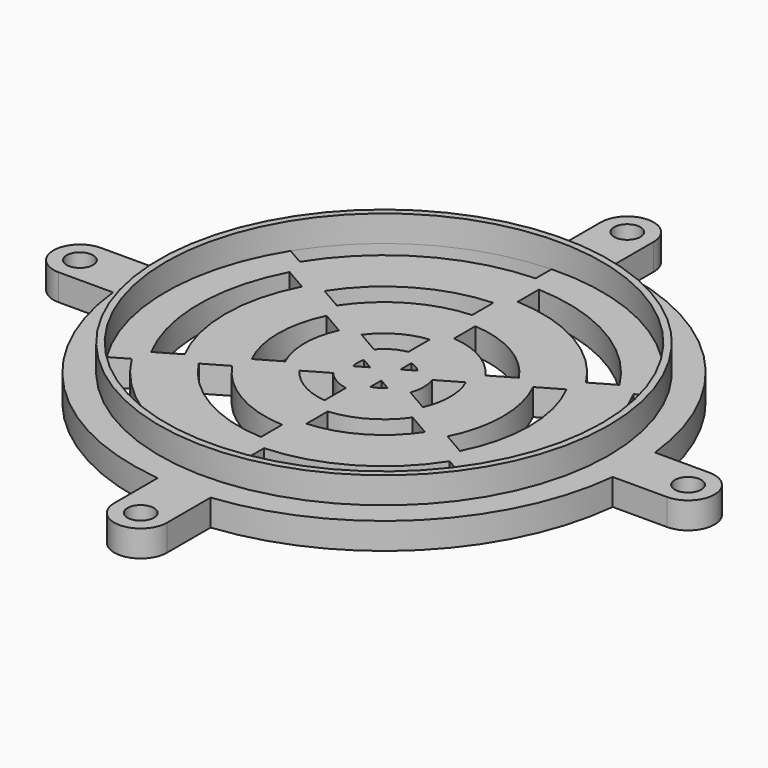
from build123d import *

# Parameters (mm, degrees)
F0_R     = 1.5875
F1_DEPTH = 3.175
F2_R     = 26.9875
F2_R_2   = 26.19375
F3_DEPTH = 3.175
F5_DEPTH = 3.175


# Not quite as in the source:
# - after a boolean that leaves OpenCascade's solid faulty, fix() repairs it


with BuildPart() as f1:
    # F0 (on Top) → F1 (new body)
    with BuildSketch(Plane.XY):
        with BuildLine():
            Line((36.5125, 3.175), (29.994929259, 3.175))
            ThreePointArc((29.994929259, 3.175), (21.3281082875, 21.3281082875), (3.175, 29.994929259))
            Line((3.175, 29.994929259), (3.175, 36.5125))
            ThreePointArc((3.175, 36.5125), (0, 39.6875), (-3.175, 36.5125))
            Line((-3.175, 36.5125), (-3.175, 29.994929259))
            ThreePointArc((-3.175, 29.994929259), (-21.3281082875, 21.3281082875), (-29.994929259, 3.175))
            Line((-29.994929259, 3.175), (-30.1625, 3.175))
            Line((-30.1625, 3.175), (-36.5125, 3.175))
            ThreePointArc((-36.5125, 3.175), (-39.6875, 0), (-36.5125, -3.175))
            Line((-36.5125, -3.175), (-30.1625, -3.175))
            Line((-30.1625, -3.175), (-29.994929259, -3.175))
            ThreePointArc((-29.994929259, -3.175), (-21.3281082875, -21.3281082875), (-3.175, -29.994929259))
            Line((-3.175, -29.994929259), (-3.175, -36.5125))
            ThreePointArc((-3.175, -36.5125), (0, -39.6875), (3.175, -36.5125))
            Line((3.175, -36.5125), (3.175, -29.994929259))
            ThreePointArc((3.175, -29.994929259), (21.3281082875, -21.3281082875), (29.994929259, -3.175))
            Line((29.994929259, -3.175), (36.5125, -3.175))
            ThreePointArc((36.5125, -3.175), (39.6875, 0), (36.5125, 3.175))
        make_face()
        with Locations((0, -36.5125)):
            Circle(F0_R, mode=Mode.SUBTRACT)
        with Locations((-36.5125, 0)):
            Circle(F0_R, mode=Mode.SUBTRACT)
        with Locations((36.5125, 0)):
            Circle(F0_R, mode=Mode.SUBTRACT)
        with Locations((0, 36.5125)):
            Circle(F0_R, mode=Mode.SUBTRACT)
    extrude(amount=F1_DEPTH)

    # F2 (on face) → F3 (join)
    with BuildSketch(Plane.XY.offset(3.175)):
        Circle(F2_R)
        Circle(F2_R_2, mode=Mode.SUBTRACT)
    extrude(amount=F3_DEPTH)

    # F4 (on face) → F5 (cut)
    with BuildSketch(Plane.XY.offset(3.175)):
        with BuildLine():
            ThreePointArc((-0.8255, 26.1807388897), (-13.096875, 22.6844529204), (-22.2604349684, 13.8052734157))
            Line((-22.2604349684, 13.8052734157), (-20.1970845335, 12.6139974867))
            ThreePointArc((-20.1970845335, 12.6139974867), (-11.90625, 20.6222299276), (-0.8255, 23.7981870318))
            Line((-0.8255, 23.7981870318), (-0.8255, 26.1807388897))
        make_face()
        with BuildLine():
            ThreePointArc((0.8255, 19.0321057624), (9.525, 16.4977839421), (16.0695370777, 10.230956852))
            Line((16.0695370777, 10.230956852), (18.8213832288, 11.8197359681))
            ThreePointArc((18.8213832288, 11.8197359681), (11.1125, 19.2474145991), (0.8255, 22.2096639945))
            Line((0.8255, 22.2096639945), (0.8255, 19.0321057624))
        make_face()
        with BuildLine():
            Line((21.0225845335, -11.1841895451), (23.0859349684, -12.375465474))
            ThreePointArc((23.0859349684, -12.375465474), (25.4049183047, -6.3798640262), (26.19375, 0))
            ThreePointArc((26.19375, 0), (25.4049183047, 6.3798640262), (23.0859349684, 12.375465474))
            Line((23.0859349684, 12.375465474), (21.0225845335, 11.1841895451))
            ThreePointArc((21.0225845335, 11.1841895451), (23.8125, 0), (21.0225845335, -11.1841895451))
        make_face()
        with BuildLine():
            Line((12.7654179102, -6.4169121723), (15.5188114324, -8.0065846636))
            ThreePointArc((15.5188114324, -8.0065846636), (17.4625, 0), (15.5188114324, 8.0065846636))
            Line((15.5188114324, 8.0065846636), (12.7654179102, 6.4169121723))
            ThreePointArc((12.7654179102, 6.4169121723), (14.2875, 0), (12.7654179102, -6.4169121723))
        make_face()
        with BuildLine():
            Line((4.4747651403, -1.6303015639), (7.2495505675, -3.2323246772))
            ThreePointArc((7.2495505675, -3.2323246772), (7.9375, 0), (7.2495505675, 3.2323246772))
            Line((7.2495505675, 3.2323246772), (4.4747651403, 1.6303015639))
            ThreePointArc((4.4747651403, 1.6303015639), (4.7625, 0), (4.4747651403, -1.6303015639))
        make_face()
        with BuildLine():
            ThreePointArc((0.8255, 9.4891609086), (4.7625, 8.248891971), (7.8051044075, 5.4594844251))
            Line((7.8051044075, 5.4594844251), (10.5625136557, 7.0514753969))
            ThreePointArc((10.5625136557, 7.0514753969), (6.35, 10.9985226281), (0.8255, 12.6731428521))
            Line((0.8255, 12.6731428521), (0.8255, 9.4891609086))
        make_face()
        with BuildLine():
            ThreePointArc((-11.9399179102, 7.846720114), (-7.14375, 12.3733379566), (-0.8255, 14.2636322863))
            Line((-0.8255, 14.2636322863), (-0.8255, 17.4429772688))
            ThreePointArc((-0.8255, 17.4429772688), (-8.73125, 15.1229686136), (-14.6933114324, 9.4363926052))
            Line((-14.6933114324, 9.4363926052), (-11.9399179102, 7.846720114))
        make_face()
        with BuildLine():
            ThreePointArc((-16.8950370777, -8.8011489104), (-19.05, 0), (-16.8950370777, 8.8011489104))
            Line((-16.8950370777, 8.8011489104), (-19.6468832288, 10.3899280264))
            ThreePointArc((-19.6468832288, 10.3899280264), (-22.225, 0), (-19.6468832288, -10.3899280264))
            Line((-19.6468832288, -10.3899280264), (-16.8950370777, -8.8011489104))
        make_face()
        with BuildLine():
            ThreePointArc((-8.6306044075, -4.0296764835), (-9.525, 0), (-8.6306044075, 4.0296764835))
            Line((-8.6306044075, 4.0296764835), (-11.3880136557, 5.6216674552))
            ThreePointArc((-11.3880136557, 5.6216674552), (-12.7, 0), (-11.3880136557, -5.6216674552))
            Line((-11.3880136557, -5.6216674552), (-8.6306044075, -4.0296764835))
        make_face()
        with BuildLine():
            ThreePointArc((-0.8255, -14.2636322863), (-7.14375, -12.3733379566), (-11.9399179102, -7.846720114))
            Line((-11.9399179102, -7.846720114), (-14.6933114324, -9.4363926052))
            ThreePointArc((-14.6933114324, -9.4363926052), (-8.73125, -15.1229686136), (-0.8255, -17.4429772688))
            Line((-0.8255, -17.4429772688), (-0.8255, -14.2636322863))
        make_face()
        with BuildLine():
            ThreePointArc((-22.2604349684, -13.8052734157), (-13.096875, -22.6844529204), (-0.8255, -26.1807388897))
            Line((-0.8255, -26.1807388897), (-0.8255, -23.7981870318))
            ThreePointArc((-0.8255, -23.7981870318), (-11.90625, -20.6222299276), (-20.1970845335, -12.6139974867))
            Line((-20.1970845335, -12.6139974867), (-22.2604349684, -13.8052734157))
        make_face()
        with BuildLine():
            ThreePointArc((16.0695370777, -10.230956852), (9.525, -16.4977839421), (0.8255, -19.0321057624))
            Line((0.8255, -19.0321057624), (0.8255, -22.2096639945))
            ThreePointArc((0.8255, -22.2096639945), (11.1125, -19.2474145991), (18.8213832288, -11.8197359681))
            Line((18.8213832288, -11.8197359681), (16.0695370777, -10.230956852))
        make_face()
        with BuildLine():
            ThreePointArc((7.8051044075, -5.4594844251), (4.7625, -8.248891971), (0.8255, -9.4891609086))
            Line((0.8255, -9.4891609086), (0.8255, -12.6731428521))
            ThreePointArc((0.8255, -12.6731428521), (6.35, -10.9985226281), (10.5625136557, -7.0514753969))
            Line((10.5625136557, -7.0514753969), (7.8051044075, -5.4594844251))
        make_face()
        with BuildLine():
            ThreePointArc((-0.8255, -4.6904110694), (-2.38125, -4.1244459855), (-3.6492651403, -3.0601095055))
            Line((-3.6492651403, -3.0601095055), (-6.4240505675, -4.6621326189))
            ThreePointArc((-6.4240505675, -4.6621326189), (-3.96875, -6.8740766425), (-0.8255, -7.8944572961))
            Line((-0.8255, -7.8944572961), (-0.8255, -4.6904110694))
        make_face()
        with BuildLine():
            ThreePointArc((-3.6492651403, 3.0601095055), (-2.38125, 4.1244459855), (-0.8255, 4.6904110694))
            Line((-0.8255, 4.6904110694), (-0.8255, 7.8944572961))
            ThreePointArc((-0.8255, 7.8944572961), (-3.96875, 6.8740766425), (-6.4240505675, 4.6621326189))
            Line((-6.4240505675, 4.6621326189), (-3.6492651403, 3.0601095055))
        make_face()
        with BuildLine():
            Line((0.8255, 1.4298079416), (2.2423170542, 2.2478076493))
            ThreePointArc((2.2423170542, 2.2478076493), (1.5875, 2.749630657), (0.8255, 3.065807357))
            Line((0.8255, 3.065807357), (0.8255, 1.4298079416))
        make_face()
        with BuildLine():
            Line((0.8255, -1.4298079416), (0.8255, -3.065807357))
            ThreePointArc((0.8255, -3.065807357), (1.5875, -2.749630657), (2.2423170542, -2.2478076493))
            Line((2.2423170542, -2.2478076493), (0.8255, -1.4298079416))
        make_face()
        with BuildLine():
            Line((-1.651, 0), (-3.0678170542, 0.8179997077))
            ThreePointArc((-3.0678170542, 0.8179997077), (-3.175, 0), (-3.0678170542, -0.8179997077))
            Line((-3.0678170542, -0.8179997077), (-1.651, 0))
        make_face()
    extrude(amount=-F5_DEPTH, mode=Mode.SUBTRACT)

    add(f1.part.fix(), mode=Mode.REPLACE)


solid = f1.part
